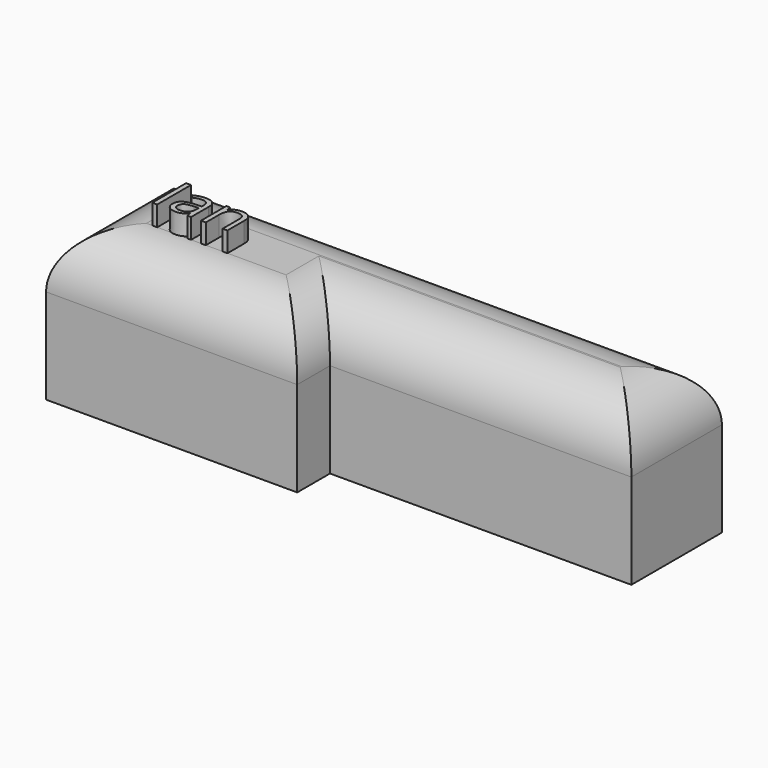
from build123d import *

# Parameters (mm, degrees)
F0_W         = 76.2
F0_H         = 28.6236796528
F1_DEPTH     = 38.1
F2_R         = 14.1038356314
F3_TEXT_SIZE = 14.9653546816
F4_DEPTH     = 5.08


# Not quite as in the source:
# - Text() gives the source's letters only with a copy of the font that has no kerning and outlines rounded to 1/6400 em; it was checked with that copy


with BuildPart() as f1:
    # F0 (on Top) → F1 (new body)
    with BuildSketch(Plane.XY):
        with Locations((38.1, -14.3118398264)):
            Rectangle(F0_W, F0_H)
        Polygon((0, -38.9827266335), (0, -28.6236796528), (0, 0), (-63.5, 0), (-63.5, -38.9827266335), align=None)
    extrude(amount=F1_DEPTH)

    # F2
    f2_edges = [f1.edges().sort_by_distance(p)[0] for p in [
        (6.35, 0, 38.1),
        (-63.5, -19.491363, 38.1),
        (-31.75, -38.982727, 38.1),
        (38.1, -28.62368, 38.1),
        (76.2, -14.31184, 38.1),
        (0, -33.803203, 38.1),
    ]]
    fillet(f2_edges, radius=F2_R)

    # F3 (on face) → F4 (join)
    with BuildSketch(Plane.XY.offset(38.1)):
        with Locations((-49.3961643686, -24.8788910022)):
            Text('Ian', F3_TEXT_SIZE, font='Open Sans', text_align=(TextAlign.LEFT, TextAlign.BOTTOM))
    extrude(amount=F4_DEPTH)


solid = f1.part
